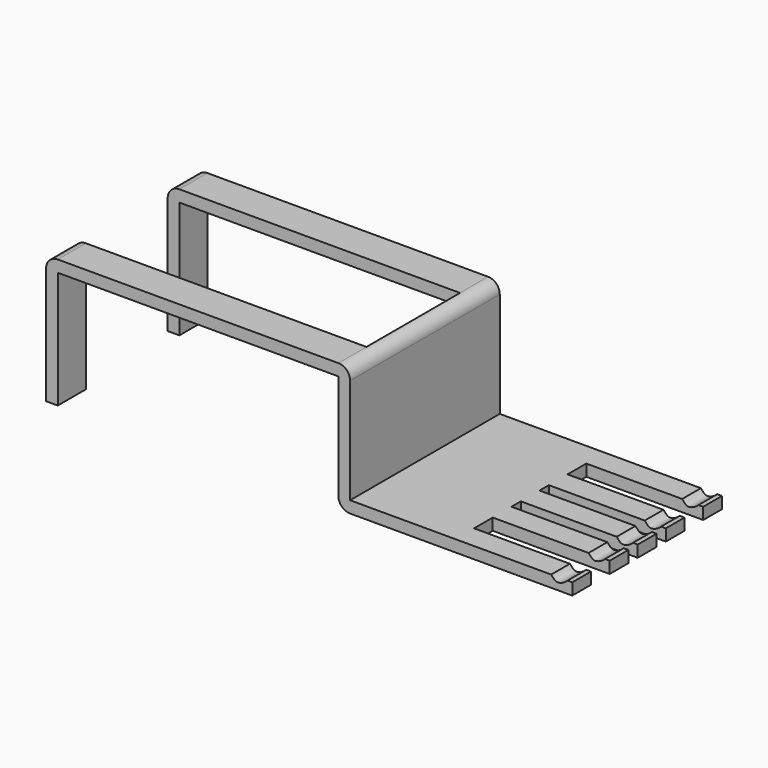
from build123d import *

# Parameters (mm, degrees)
F0_W      = 50
F0_H      = 10
F1_DEPTH  = 5
F0_W_2    = 5
F0_H_2    = 80
F2_DEPTH  = 55
F3_W      = 15
F3_H      = 5
F4_DEPTH  = 125
F6_W      = 5
F6_H      = 15
F5_W      = 5
F5_H      = 15
F7_DEPTH  = 50
F8_R      = 4.99999
F10_DEPTH = 80.001


# Not quite as in the source:
# - a fillet or chamfer is up to 0.001 mm smaller than in the source, because OpenCascade refuses the exact size


with BuildPart() as f1:
    # F0 (on Top) → F1 (new body)
    with BuildSketch(Plane.XY):
        Polygon((59.8684251308, 39.4171364857), (14.8684251308, 39.4171364857), (14.8684251308, -40.5828635143), (59.8684251308, -40.5828635143), (59.8684251308, -30.5828635143), (59.8684251308, -20.5828635143), (59.8684251308, -10.5828635143), (59.8684251308, -5.5828635143), (59.8684251308, 4.4171364857), (59.8684251308, 9.4171364857), (59.8684251308, 19.4171364857), (59.8684251308, 29.4171364857), align=None)
        with Locations((84.8684251308, -0.5828635143)):
            Rectangle(F0_W, F0_H)
        with Locations((84.8684251308, -35.5828635143)):
            Rectangle(F0_W, F0_H)
        with Locations((84.8684251308, 14.4171364857)):
            Rectangle(F0_W, F0_H)
        with Locations((84.8684251308, 34.4171364857)):
            Rectangle(F0_W, F0_H)
        with Locations((84.8684251308, -15.5828635143)):
            Rectangle(F0_W, F0_H)
    extrude(amount=F1_DEPTH)

    # F0 (on Top) → F2 (join)
    with BuildSketch(Plane.XY):
        with Locations((12.3684251308, -0.5828635143)):
            Rectangle(F0_W_2, F0_H_2)
    extrude(amount=F2_DEPTH)

    # F3 (on face) → F4 (join)
    with BuildSketch(Plane(origin=(9.8684251308, 0, 0), x_dir=(0, -1, 0), z_dir=(-1, 0, 0))):
        with Locations((-31.9171364857, 52.5)):
            Rectangle(F3_W, F3_H)
        with Locations((33.0828635143, 52.5)):
            Rectangle(F3_W, F3_H)
    extrude(amount=F4_DEPTH)

    # F6 (on face) + F5 (on face) → F7 (join)
    with BuildSketch(Plane(origin=(0, 0, 50), x_dir=(1, 0, 0), z_dir=(0, 0, -1))):
        with Locations((-112.6315748692, 33.0828635143)):
            Rectangle(F6_W, F6_H)
    with BuildSketch(Plane(origin=(0, 0, 50), x_dir=(1, 0, 0), z_dir=(0, 0, -1))):
        with Locations((-112.6315748692, -31.9171364857)):
            Rectangle(F5_W, F5_H)
    extrude(amount=F7_DEPTH)

    # F8 (radius 5 in the source; OpenCascade refuses exactly that, so slightly less here)
    f8_edges = [f1.edges().sort_by_distance(p)[0] for p in [
        (-115.131575, 31.917136, 55),
        (-115.131575, -33.082864, 55),
        (9.868425, -0.582864, 0),
        (14.868425, -0.582864, 55),
    ]]
    fillet(f8_edges, radius=F8_R)

    # F9 (on face) → F10 (cut, through all)
    with BuildSketch(Plane.XZ.offset(40.5828635143)):
        with BuildLine():
            add(Edge.make_bspline(
                [(107.8684251308, 5), (106.7611965953, 3.8240237002), (103.011923181, 1.9991854383), (101.7375563624, 4.0782074875), (100.8684251308, 5)],
                knots=[0, 0, 0, 0, 0.5536142678, 1, 1, 1, 1], degree=3))
            Line((107.8684251308, 5), (100.8684251308, 5))
        make_face()
    extrude(amount=-F10_DEPTH, mode=Mode.SUBTRACT)


solid = f1.part
